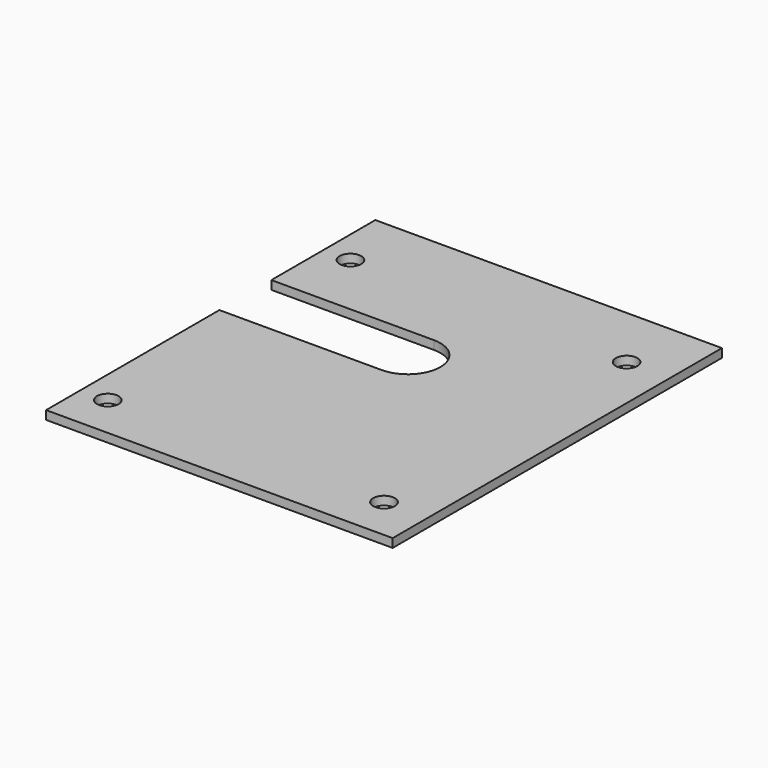
from build123d import *

# Parameters (mm, degrees)
F0_W     = 32
F0_H     = 38
F1_DEPTH = 0.8
F2_R     = 1
F2_W     = 18
F2_H     = 6
F3_DEPTH = 0.8
F4_R     = 2.99999


# Not quite as in the source:
# - a fillet or chamfer is up to 0.001 mm smaller than in the source, because OpenCascade refuses the exact size


with BuildPart() as f1:
    # F0 (on Top) → F1 (new body)
    with BuildSketch(Plane.XY):
        with Locations((-9.963327945, 1.2697370127)):
            Rectangle(F0_W, F0_H)
    extrude(amount=F1_DEPTH)

    # F2 (on face) → F3 (cut, through all)
    with BuildSketch(Plane(origin=(0, 0, 0), x_dir=(1, 0, 0), z_dir=(0, 0, -1))):
        with Locations((-23.463327945, 13.7302629873)):
            Circle(F2_R)
        with Locations((-23.463327945, -14.2697370127)):
            Circle(F2_R)
        with Locations((2.036672055, 13.7302629873)):
            Circle(F2_R)
        with Locations((2.036672055, -14.2697370127)):
            Circle(F2_R)
        with Locations((-16.963327945, -5.2697370127)):
            Rectangle(F2_W, F2_H)
    extrude(amount=-F3_DEPTH, mode=Mode.SUBTRACT)

    # F4 (radius 3 in the source; OpenCascade refuses exactly that, so slightly less here)
    f4_edges = [f1.edges().sort_by_distance(p)[0] for p in [
        (-7.963328, 8.269737, 0.4),
        (-7.963328, 2.269737, 0.4),
    ]]
    fillet(f4_edges, radius=F4_R)


solid = f1.part
